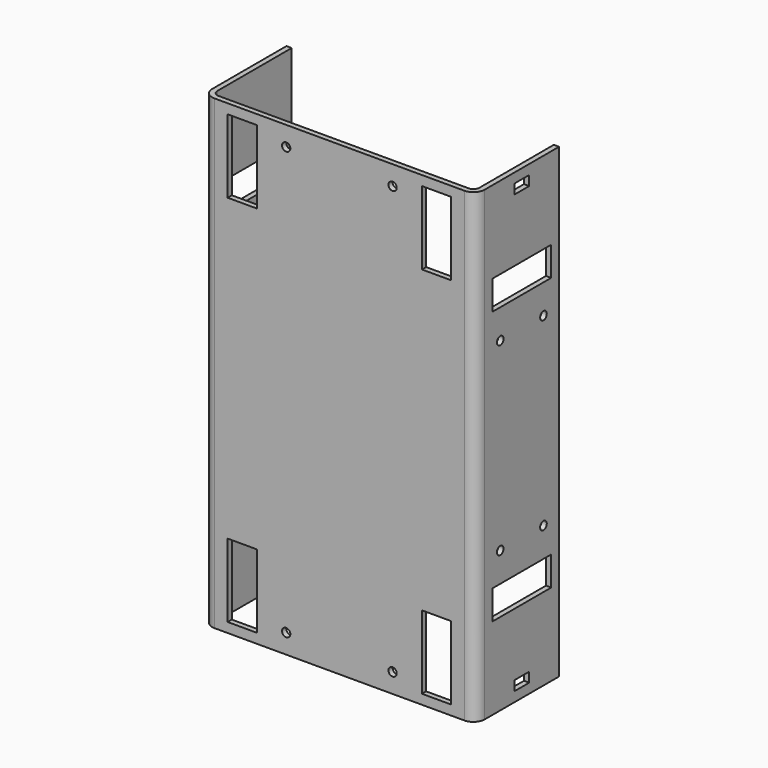
from build123d import *

# Parameters (mm, degrees)
F1_DEPTH = 152.4
F2_R     = 1.98374
F3_R     = 3.69316
F4_W     = 9.5329248
F4_H     = 24
F4_R     = 1.35255
F5_DEPTH = 1.70942
F6_W     = 24
F6_H     = 9.5329248
F6_R     = 1.35255
F7_DEPTH = 89.0613408
F8_W     = 6
F8_H     = 3.175
F9_DEPTH = 1.70942


with BuildPart() as f1:
    # F0 (on Top) → F1 (new body)
    with BuildSketch(Plane.XY):
        Polygon((0, 32.3337428), (0, 0), (-85.6425008, 0), (-85.6425008, 32.3337428), (-87.3519208, 32.3337428), (-87.3519208, -1.70942), (1.70942, -1.70942), (1.70942, 32.3337428), align=None)
    extrude(amount=F1_DEPTH)

    # F2
    f2_edges = [f1.edges().sort_by_distance(p)[0] for p in [
        (0, 0, 76.2),
        (-85.642501, 0, 76.2),
    ]]
    fillet(f2_edges, radius=F2_R)

    # F3
    f3_edges = [f1.edges().sort_by_distance(p)[0] for p in [
        (1.70942, -1.70942, 76.2),
        (-87.351921, -1.70942, 76.2),
    ]]
    fillet(f3_edges, radius=F3_R)

    # F4 (on face) → F5 (cut, through all)
    with BuildSketch(Plane(origin=(0, 0, 0), x_dir=(-1, 0, 0), z_dir=(0, 1, 0))):
        with Locations((74.5712504, 15.175)):
            Rectangle(F4_W, F4_H)
        with Locations((11.0712504, 15.175)):
            Rectangle(F4_W, F4_H)
        with Locations((11.0712504, 137.225)):
            Rectangle(F4_W, F4_H)
        with Locations((74.5712504, 137.225)):
            Rectangle(F4_W, F4_H)
        with Locations((60.20308, 6.35)):
            Circle(F4_R)
        with Locations((25.4394208, 6.35)):
            Circle(F4_R)
        with Locations((25.4394208, 146.05)):
            Circle(F4_R)
        with Locations((60.20308, 146.05)):
            Circle(F4_R)
    extrude(amount=-F5_DEPTH, mode=Mode.SUBTRACT)

    # F6 (on face) → F7 (cut, through all)
    with BuildSketch(Plane(origin=(-87.3519208, 0, 0), x_dir=(0, -1, 0), z_dir=(-1, 0, 0))):
        with Locations((-17.15874, 31.6544706)):
            Rectangle(F6_W, F6_H)
        with Locations((-17.15874, 120.7455294)):
            Rectangle(F6_W, F6_H)
        with Locations((-25.98374, 46.022641)):
            Circle(F6_R)
        with Locations((-25.98374, 106.377359)):
            Circle(F6_R)
        with Locations((-8.33374, 106.377359)):
            Circle(F6_R)
        with Locations((-8.33374, 46.022641)):
            Circle(F6_R)
    extrude(amount=-F7_DEPTH, mode=Mode.SUBTRACT)

    # F8 (on face) → F9 (cut, through all)
    with BuildSketch(Plane.YZ.offset(1.70942)):
        with Locations((17.1587414, 4.7625)):
            Rectangle(F8_W, F8_H)
        with Locations((17.1587414, 147.6375)):
            Rectangle(F8_W, F8_H)
    extrude(amount=-F9_DEPTH, mode=Mode.SUBTRACT)


solid = f1.part
